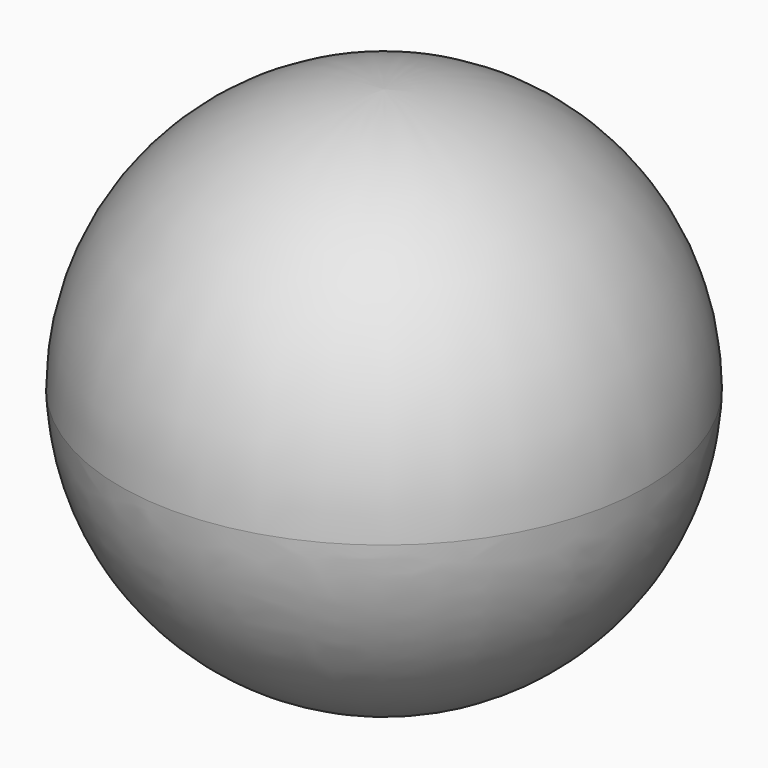
from build123d import *

# Parameters (mm, degrees)
F0_R     = 45.214458384
F1_DEPTH = 88.9
F2_R     = 45.212


# Not quite as in the source:
# - a fillet or chamfer that OpenCascade refuses, or shapes differently, is made with other operations: its cross-section is extruded or revolved along the edge and cut away or added


with BuildPart() as f1:
    # F0 (on Top) → F1 (new body)
    with BuildSketch(Plane.XY):
        Circle(F0_R)
    extrude(amount=F1_DEPTH)

    # F2
    f2_edges = [f1.edges().sort_by_distance(p)[0] for p in [
        (-45.214458, 0, 88.9),
    ]]
    fillet(f2_edges, radius=F2_R)

    # F3: fillet of radius 45.212 on 1 edges, made by hand

    # F3_s1 → F3_t2 (revolve, cut)
    with BuildSketch(Plane.XZ):
        with BuildLine():
            ThreePointArc((45.214458384, 43.688), (31.4544287444, 12.7079384692), (0.0281510775, 0))
            Line((0.0281510775, 0), (0.0281510775, -0.90424))
            Line((0.0281510775, -0.90424), (45.214458384, -0.90424))
            Line((45.214458384, -0.90424), (46.118698384, 0))
            ThreePointArc((46.118698384, 0), (46.118698384, 21.844), (46.1181845301, 43.65752))
            Line((46.1181845301, 43.65752), (45.214458384, 43.688))
        make_face()
    revolve(axis=Axis((0, 0, 0), (0, 0, 1)), mode=Mode.SUBTRACT)


solid = f1.part
